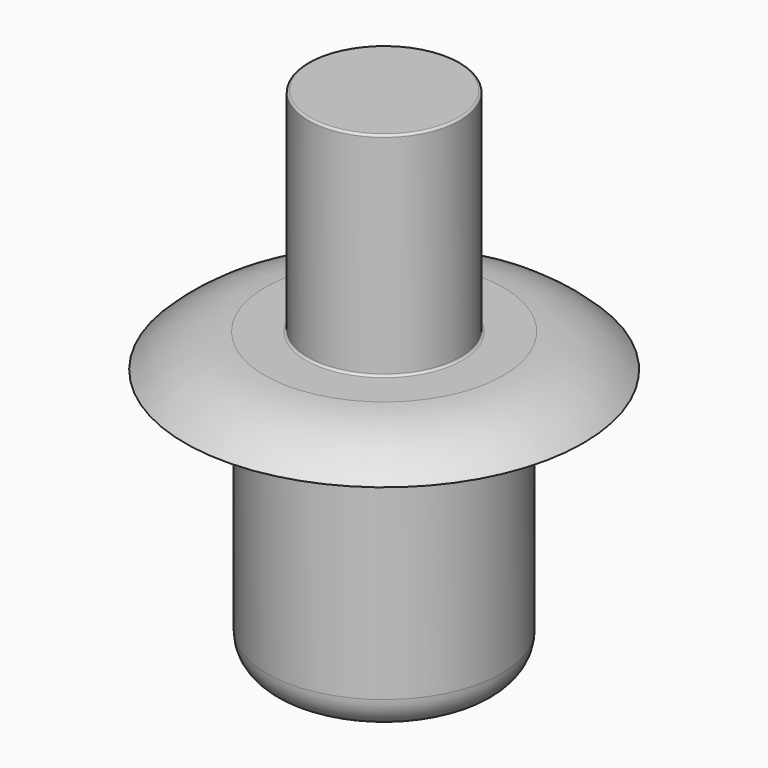
from build123d import *

# Parameters (mm, degrees)
F0_R     = 5.25
F1_DEPTH = 11.7
F2_R     = 8.9
F3_DEPTH = 1.5
F4_R     = 3.4
F5_DEPTH = 9.5
F7_R     = 0.0965685425
F8_R     = 3.4
F9_DEPTH = 11.8
F10_R    = 1.4485281374


# Not quite as in the source:
# - a fillet or chamfer that OpenCascade refuses, or shapes differently, is made with other operations: its cross-section is extruded or revolved along the edge and cut away or added


with BuildPart() as f1:
    # F0 (on Top) → F1 (new body)
    with BuildSketch(Plane.XY):
        Circle(F0_R)
    extrude(amount=F1_DEPTH)

    # F2 (on face) → F3 (join)
    with BuildSketch(Plane.XY.offset(11.7)):
        Circle(F2_R)
    extrude(amount=F3_DEPTH)

    # F4 (on face) → F5 (join)
    with BuildSketch(Plane.XY.offset(13.2)):
        Circle(F4_R)
    extrude(amount=F5_DEPTH)

    # F6: fillet of radius 5 on 1 edges, made by hand

    # F6_s1 → F6_t2 (revolve, cut)
    with BuildSketch(Plane.XZ):
        with BuildLine():
            ThreePointArc((8.9, 11.7), (7.2657774588, 12.8097722286), (5.3292857857, 13.2))
            Line((5.3292857857, 13.2), (8.9, 13.2))
            Line((8.9, 13.2), (8.9, 11.7))
        make_face()
    revolve(axis=Axis((0, 0, 13.2), (0, 0, 1)), mode=Mode.SUBTRACT)

    # F7
    f7_edges = [f1.edges().sort_by_distance(p)[0] for p in [
        (3.4, 0, 17.95),
        (-3.4, 0, 13.2),
        (-3.4, 0, 22.7),
    ]]
    fillet(f7_edges, radius=F7_R)

    # F8 (on face) → F9 (cut)
    with BuildSketch(Plane(origin=(0, 0, 0), x_dir=(1, 0, 0), z_dir=(0, 0, -1))):
        Circle(F8_R)
    extrude(amount=-F9_DEPTH, mode=Mode.SUBTRACT)

    # F10
    f10_edges = [f1.edges().sort_by_distance(p)[0] for p in [
        (-5.25, 0, 0),
    ]]
    fillet(f10_edges, radius=F10_R)


solid = f1.part
